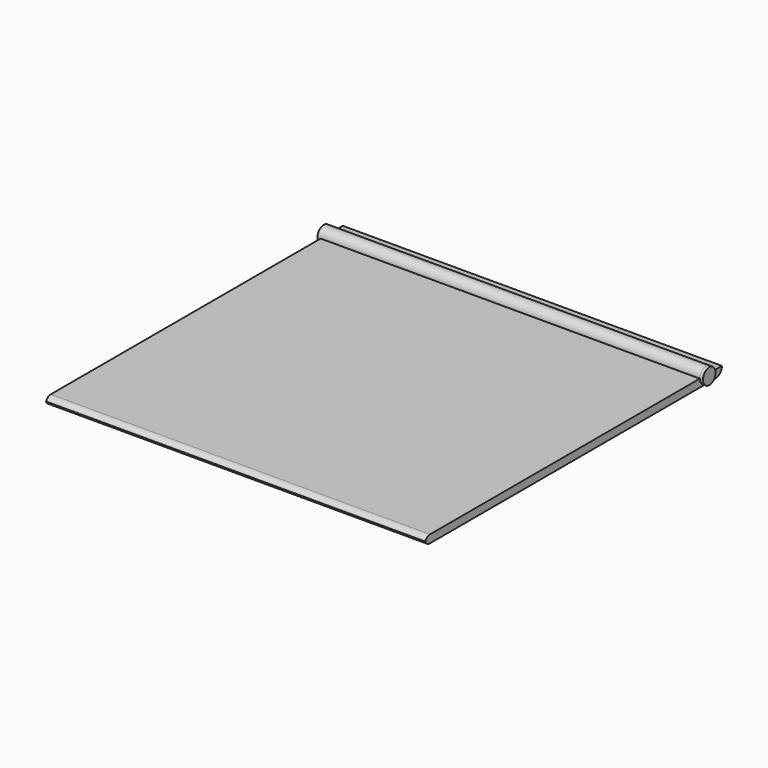
from build123d import *

# Parameters (mm, degrees)
F0_W          = 304.8
F0_H          = 298.45
F1_DEPTH      = 6.35
F2_R          = 6.34999
F3_R          = 6.35
F4_DEPTH      = 2.54
F4_DEPTH_BACK = 307.34
F5_T1_DEPTH   = 330.2


# Not quite as in the source:
# - a fillet or chamfer that OpenCascade refuses, or shapes differently, is made with other operations: its cross-section is extruded or revolved along the edge and cut away or added
# - a fillet or chamfer is up to 0.001 mm smaller than in the source, because OpenCascade refuses the exact size


with BuildPart() as f1:
    # F0 (on Top) → F1 (new body)
    with BuildSketch(Plane.XY):
        Rectangle(F0_W, F0_H)
    extrude(amount=F1_DEPTH)

    # F2 (radius 6.35 in the source; OpenCascade refuses exactly that, so slightly less here)
    f2_edges = [f1.edges().sort_by_distance(p)[0] for p in [
        (0, 149.225, 0),
    ]]
    fillet(f2_edges, radius=F2_R)

    # F3 (on face) → F4 (join, two sides)
    with BuildSketch(Plane.YZ.offset(152.4)) as f4_sk:
        with Locations((133.35, 6.35)):
            Circle(F3_R)
    extrude(amount=F4_DEPTH)
    extrude(f4_sk.sketch, amount=-F4_DEPTH_BACK)

    # F5: fillet of radius 5.08 on 2 edges, made by hand

    # F5_s2 → F5_t1 (cut)
    with BuildSketch(Plane.YZ.offset(-165.1)):
        with BuildLine():
            ThreePointArc((-144.145, 0), (-147.7371024484, 1.4878975516), (-149.225, 5.08))
            Line((-149.225, 5.08), (-149.225, 0))
            Line((-149.225, 0), (-144.145, 0))
        make_face()
        with BuildLine():
            ThreePointArc((-144.145, 6.35), (-147.7371024484, 4.8621024484), (-149.225, 1.27))
            Line((-149.225, 1.27), (-149.225, 6.35))
            Line((-149.225, 6.35), (-144.145, 6.35))
        make_face()
    extrude(amount=F5_T1_DEPTH, mode=Mode.SUBTRACT)


solid = f1.part
